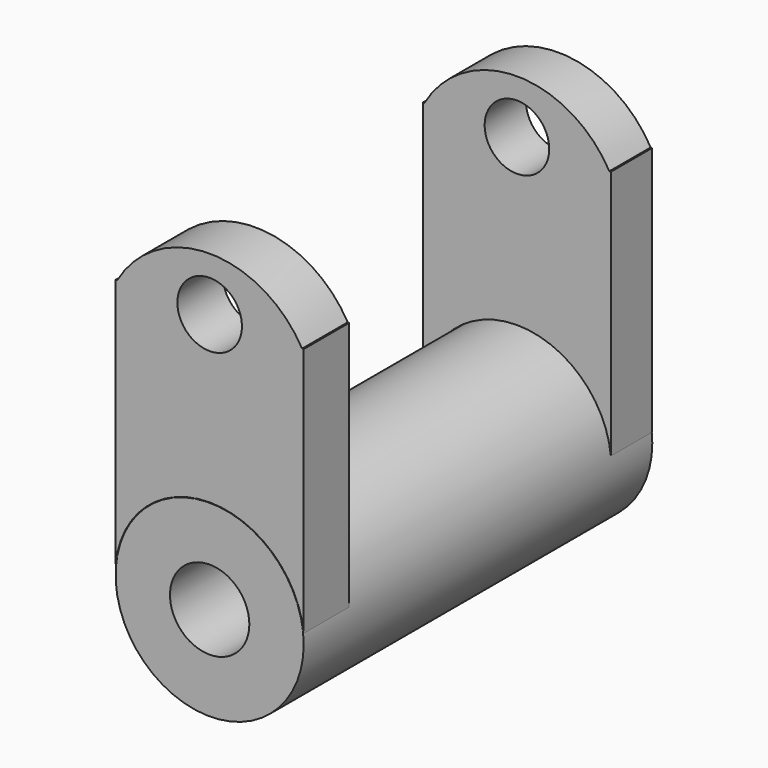
from build123d import *

# Parameters (mm, degrees)
F0_R     = 27.4116856275
F0_R_2   = 11.5663237111
F1_DEPTH = 127
F3_DEPTH = 127
F4_W     = 95.3267142177
F4_H     = 18.8548341393
F4_H_2   = 72.9184712529
F5_DEPTH = 54.7957877316


# Not quite as in the source:
# - a feature of the source that left no trace in its solid (it failed there, or was rolled back) is left out


with BuildPart() as f1:
    # F0 (on Front) → F1 (new body)
    with BuildSketch(Plane.XZ):
        Circle(F0_R)
        Circle(F0_R_2, mode=Mode.SUBTRACT)
    extrude(amount=F1_DEPTH)


with BuildPart() as f3:
    # F2 (on Front) → F3 (new body)
    with BuildSketch(Plane.XZ):
        with BuildLine():
            Line((-26.9458102859, 75.7313892245), (-27.3831021041, 75.7313892245))
            Line((-27.3831021041, 75.7313892245), (-27.3831021041, 74.9398508998))
            ThreePointArc((-27.3831021041, 74.9398508998), (-27.1673390968, 75.3372127448), (-26.9458102859, 75.7313892245))
        make_face()
        with BuildLine():
            Line((-9.4129424542, 75.7313892245), (-26.9458102859, 75.7313892245))
            ThreePointArc((-26.9458102859, 75.7313892245), (-27.1673390968, 75.3372127448), (-27.3831021041, 74.9398508998))
            Line((-27.3831021041, 74.9398508998), (-27.3831021041, 2.8129179717))
            ThreePointArc((-27.3831021041, 2.8129179717), (0, 27.5272008813), (27.3831021041, 2.8129179717))
            Line((27.3831021041, 2.8129179717), (27.3831021041, 74.9398508998))
            ThreePointArc((27.3831021041, 74.9398508998), (27.1673390968, 75.3372127448), (26.9458102859, 75.7313892245))
            Line((26.9458102859, 75.7313892245), (9.4129424542, 75.7313892245))
            ThreePointArc((9.4129424542, 75.7313892245), (0, 66.3184467703), (-9.4129424542, 75.7313892245))
        make_face()
        with BuildLine():
            ThreePointArc((26.9458102859, 75.7313892245), (0, 91.3659351286), (-26.9458102859, 75.7313892245))
            Line((-26.9458102859, 75.7313892245), (-9.4129424542, 75.7313892245))
            ThreePointArc((-9.4129424542, 75.7313892245), (0, 85.1443316787), (9.4129424542, 75.7313892245))
            Line((9.4129424542, 75.7313892245), (26.9458102859, 75.7313892245))
        make_face()
        with BuildLine():
            Line((27.3831021041, 75.7313892245), (26.9458102859, 75.7313892245))
            ThreePointArc((26.9458102859, 75.7313892245), (27.1673390968, 75.3372127448), (27.3831021041, 74.9398508998))
            Line((27.3831021041, 74.9398508998), (27.3831021041, 75.7313892245))
        make_face()
    extrude(amount=F3_DEPTH)

    # F4 (on face) → F5 (cut, through all)
    with BuildSketch(Plane.YZ.offset(27.3831021041)):
        with Locations((-62.7153925598, 85.1588062942)):
            Rectangle(F4_W, F4_H)
        with Locations((-62.7153925598, 39.2721535981)):
            Rectangle(F4_W, F4_H_2)
    extrude(amount=-F5_DEPTH, mode=Mode.SUBTRACT)


solid = Compound([f1.part, f3.part])
